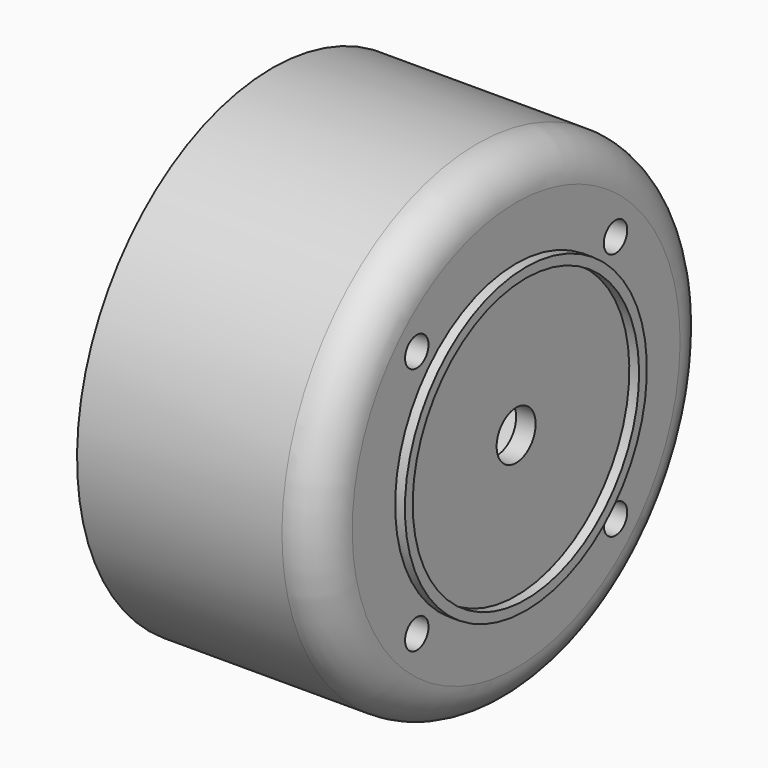
from build123d import *

# Parameters (mm, degrees)
F2_R            = 2.5
F3_DEPTH        = 25.001
F2_R_2          = 1.5
F4_DEPTH        = 25.001
F4_COPIES_COUNT = 4


# Not quite as in the source:
# - a pattern or mirror of a feature is missing from the dataset's text; its kind, count and spacing are read off the source's solid


with BuildPart() as f1:
    # F0 (on Front) → F1 (revolve)
    with BuildSketch(Plane.XZ):
        with BuildLine():
            Line((0, 25), (0, 23.5))
            Line((0, 23.5), (20.5, 23.5))
            ThreePointArc((20.5, 23.5), (22.267766953, 22.767766953), (23, 21))
            Line((23, 21), (23, 0))
            Line((23, 0), (25, 0))
            Line((25, 0), (25, 14.5))
            Line((25, 14.5), (26, 14.5))
            Line((26, 14.5), (26, 15.5))
            Line((26, 15.5), (25, 15.5))
            Line((25, 15.5), (25, 21))
            ThreePointArc((25, 21), (23.8284271247, 23.8284271247), (21, 25))
            Line((21, 25), (0, 25))
        make_face()
    revolve(axis=Axis((24, 0, 0), (-1, 0, 0)))

    # F2 (on face) → F3 (cut, through all)
    with BuildSketch(Plane.YZ.offset(25)):
        Circle(F2_R)
    extrude(amount=-F3_DEPTH, mode=Mode.SUBTRACT)

    # F2 (on face) → F4 (cut, through all)
    with BuildSketch(Plane.YZ.offset(25)):
        with Locations((-12.7279220614, 12.7279220614)):
            Circle(F2_R_2)
    f4 = extrude(amount=-F4_DEPTH, mode=Mode.SUBTRACT)

    # F4_copies: F4 ×4 about axis
    f4_copies_axis = Axis((0, 0, 0), (1, 0, 0))
    for i in range(1, F4_COPIES_COUNT):
        add(f4.rotate(f4_copies_axis, i * 360 / F4_COPIES_COUNT), mode=Mode.SUBTRACT)


solid = f1.part
